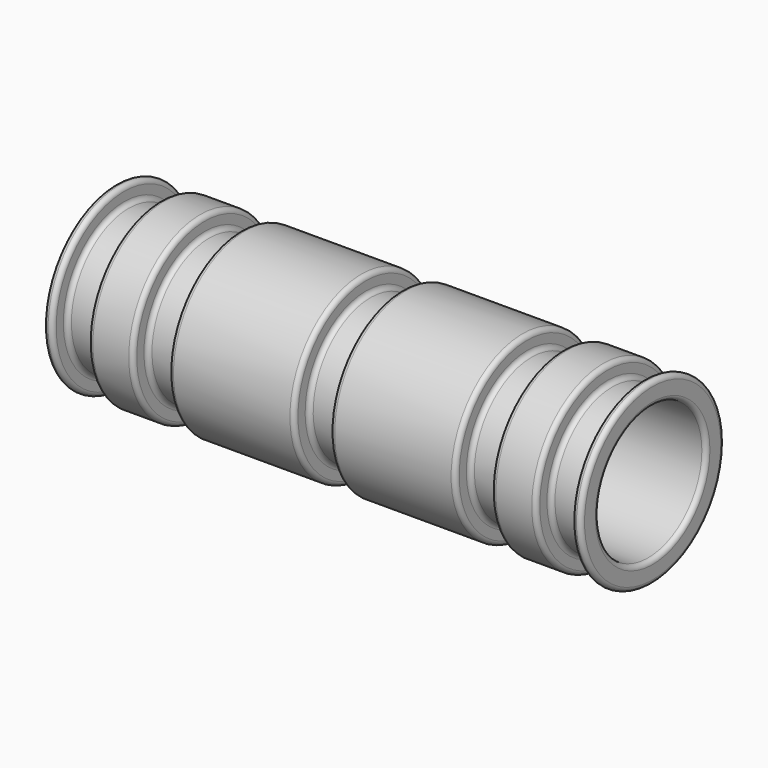
from build123d import *

# Parameters (mm, degrees)
F0_R     = 25.4
F0_R_2   = 19.05
F1_DEPTH = 76.2
F2_W     = 10.16
F2_H     = 20.32
F4_R     = 1.26999


# Not quite as in the source:
# - a fillet or chamfer is up to 0.001 mm smaller than in the source, because OpenCascade refuses the exact size


with BuildPart() as f1:
    # F0 (on Right) → F1 (new body, symmetric)
    with BuildSketch(Plane.YZ):
        Circle(F0_R)
        Circle(F0_R_2, mode=Mode.SUBTRACT)
    extrude(amount=F1_DEPTH, both=True)

    # F2 (on Front) → F3 (revolve, cut)
    with BuildSketch(Plane.XZ):
        with Locations((-68.58, 30.48)):
            Rectangle(F2_W, F2_H)
        with Locations((-45.72, 30.48)):
            Rectangle(F2_W, F2_H)
        with Locations((0, 30.48)):
            Rectangle(F2_W, F2_H)
        with Locations((45.72, 30.48)):
            Rectangle(F2_W, F2_H)
        with Locations((68.58, 30.48)):
            Rectangle(F2_W, F2_H)
    revolve(axis=Axis((-76.2, 0, 0), (1, 0, 0)), mode=Mode.SUBTRACT)

    # F4 (radius 1.27 in the source; OpenCascade refuses exactly that, so slightly less here)
    f4_edges = [f1.edges().sort_by_distance(p)[0] for p in [
        (-74.93, 25.4, 0),
        (-73.66, -25.4, 0),
        (-76.2, -25.4, 0),
        (-73.66, 0, -20.32),
        (-63.5, 0, -20.32),
        (-68.58, 0, 20.32),
        (-63.5, -25.4, 0),
        (-57.15, 25.4, 0),
        (-50.8, -25.4, 0),
        (-50.8, 0, -20.32),
        (-40.64, 0, -20.32),
        (-45.72, 0, 20.32),
        (-40.64, -25.4, 0),
        (-22.86, 25.4, 0),
        (-5.08, -25.4, 0),
        (-5.08, 0, -20.32),
        (5.08, 0, -20.32),
        (0, 0, 20.32),
        (5.08, -25.4, 0),
        (22.86, 25.4, 0),
        (40.64, -25.4, 0),
        (40.64, 0, -20.32),
        (50.8, 0, -20.32),
        (45.72, 0, 20.32),
        (50.8, -25.4, 0),
        (57.15, 25.4, 0),
        (63.5, -25.4, 0),
        (63.5, 0, -20.32),
        (73.66, 0, -20.32),
        (68.58, 0, 20.32),
        (73.66, -25.4, 0),
        (74.93, 25.4, 0),
        (76.2, -25.4, 0),
        (-76.2, -19.05, 0),
        (76.2, -19.05, 0),
    ]]
    fillet(f4_edges, radius=F4_R)


solid = f1.part
